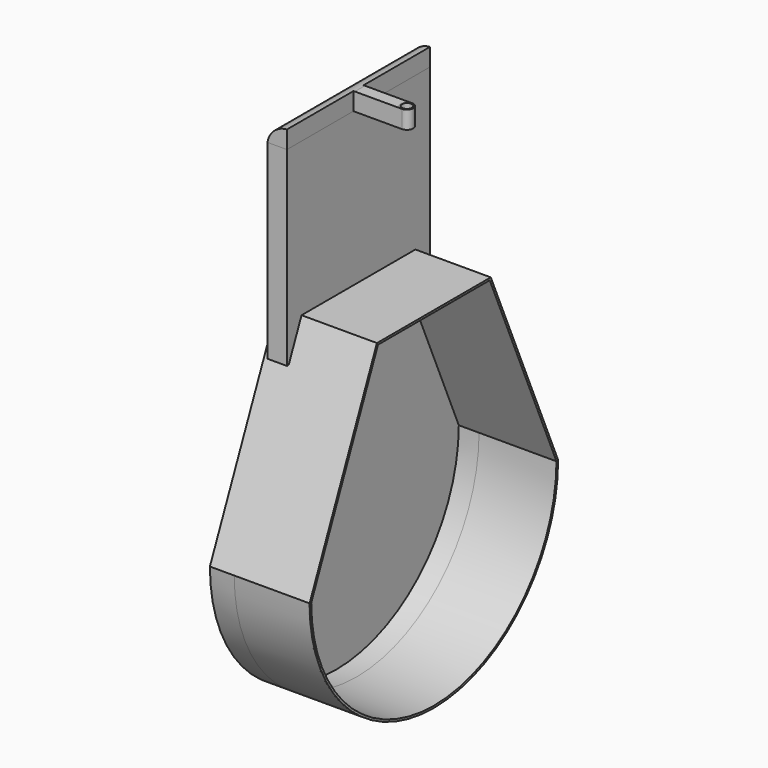
from build123d import *

# Parameters (mm, degrees)
F0_R        = 7.7629536733
F0_R_2      = 6.115
F1_DEPTH    = 21.94
F3_DEPTH    = 21.9
F4_T1_DEPTH = 349.3365371959
F7_DEPTH    = 30
F8_DEPTH    = 235
F10_DEPTH   = 93
F11_T       = -2.5
F12_DEPTH   = 92


# Not quite as in the source:
# - a fillet or chamfer that OpenCascade refuses, or shapes differently, is made with other operations: its cross-section is extruded or revolved along the edge and cut away or added


with BuildPart() as f1:
    # F0 (on Top) → F1 (new body)
    with BuildSketch(Plane.XY):
        Circle(F0_R)
        Circle(F0_R_2, mode=Mode.SUBTRACT)
    extrude(amount=F1_DEPTH)

    # F2 (on face) → F3 (join)
    with BuildSketch(Plane(origin=(0, 0, 0), x_dir=(1, 0, 0), z_dir=(0, 0, -1))):
        with BuildLine():
            ThreePointArc((0, -7.7629536733), (-7.7629536733, 0), (0, 7.7629536733))
            Line((0, 7.7629536733), (-59.79, 7.7629536733))
            Line((-59.79, 7.7629536733), (-59.79, 110.3249713778))
            Line((-59.79, 110.3249713778), (-83.8307887316, 110.3249713778))
            Line((-83.8307887316, 110.3249713778), (-83.8307887316, 0))
            Line((-83.8307887316, 0), (-83.8307887316, -110.3249713778))
            Line((-83.8307887316, -110.3249713778), (-59.79, -110.3249713778))
            Line((-59.79, -110.3249713778), (-59.79, -7.7629536733))
            Line((-59.79, -7.7629536733), (0, -7.7629536733))
        make_face()
    extrude(amount=-F3_DEPTH)

    # F4: fillet of radius 26.0735064736 on 1 edges, made by hand

    # F4_s2 → F4_t1 (cut)
    with BuildSketch(Plane.XZ.offset(-174.668268598)):
        with BuildLine():
            ThreePointArc((-58.0934698435, 21.9), (-74.9903599682, 15.6840574239), (-83.8307887316, 0))
            Line((-83.8307887316, 0), (-83.8307887316, 21.9))
            Line((-83.8307887316, 21.9), (-58.0934698435, 21.9))
        make_face()
    extrude(amount=F4_T1_DEPTH, mode=Mode.SUBTRACT)


with BuildPart() as f7:
    # F6 (on face) → F7 (new body)
    with BuildSketch(Plane.YZ.offset(-59.79)):
        with BuildLine():
            Line((-87.7716502015, -189.0654966483), (-191.6043754912, -429.56122756))
            ThreePointArc((-191.6043754912, -429.56122756), (0, -621.1656030512), (191.6043754912, -429.56122756))
            Line((191.6043754912, -429.56122756), (87.7716502015, -189.0654966483))
            Line((87.7716502015, -189.0654966483), (-87.7716502015, -189.0654966483))
        make_face()
    extrude(amount=-F7_DEPTH)

    # F9 (on face) → F10 (join)
    with BuildSketch(Plane.YZ.offset(-59.79)):
        with BuildLine():
            Line((-87.7716502015, -189.0654966483), (-191.6043754912, -429.56122756))
            ThreePointArc((-191.6043754912, -429.56122756), (0, -621.0952325876), (191.6043754912, -429.56122756))
            Line((191.6043754912, -429.56122756), (87.7716502015, -189.0654966483))
            Line((87.7716502015, -189.0654966483), (-87.7716502015, -189.0654966483))
        make_face()
    extrude(amount=F10_DEPTH)

    # F11
    f11_openings = [f7.faces().sort_by_distance(p)[0] for p in [
        (33.21, 0, -410.391358),
    ]]
    offset(amount=F11_T, openings=f11_openings, kind=Kind.INTERSECTION)


with BuildPart() as f8:
    # F5 (on face) → F8 (new body)
    with BuildSketch(Plane(origin=(0, 0, 0), x_dir=(1, 0, 0), z_dir=(0, 0, -1))):
        Polygon((-83.8307887316, 110.3249713778), (-83.8307887316, -110.3249713778), (-59.79, -110.3249713778), (-59.79, -7.7629536733), (-59.79, 7.7629536733), (-59.79, 110.3249713778), align=None)
    extrude(amount=F8_DEPTH)


with BuildPart() as f12:
    # F10_face (on face) → F12 (new body)
    with BuildSketch(Plane(origin=(-59.79, 4e-10, -580.0199905498), x_dir=(0, 1, 0), z_dir=(1, 0, 0))):
        with BuildLine():
            ThreePointArc((-191.6043754916, 150.4587629897), (-4e-10, -41.1456125014), (191.6043754908, 150.4587629897))
            ThreePointArc((191.6043754908, 150.4587629897), (-4e-10, -41.0752420379), (-191.6043754916, 150.4587629897))
        make_face()
    extrude(amount=F12_DEPTH)


solid = Compound([f1.part, f7.part, f8.part, f12.part])
